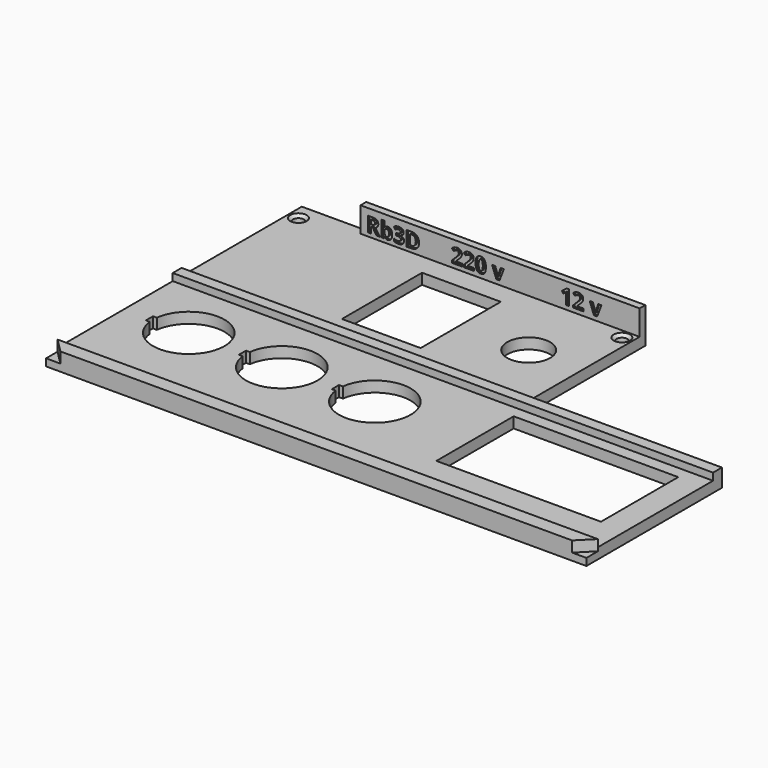
from build123d import *

# Parameters (mm, degrees)
F0_W         = 46
F0_H         = 27
F0_R         = 1.5
F0_W_2       = 22
F0_H_2       = 28
F0_R_2       = 6
F1_DEPTH     = 2
F2_DEPTH     = 10
F3_TEXT_SIZE = 5.7983598792
F4_DEPTH     = 0.5
F5_W         = 46
F5_H         = 27
F5_R         = 1.5
F5_W_2       = 22
F5_H_2       = 28
F5_R_2       = 6
F6_DEPTH     = 1
F7_SIZE      = 0.8
F9_DEPTH     = 2


# Not quite as in the source:
# - Text() gives the source's letters only with a copy of the font that has no kerning and outlines rounded to 1/6400 em; it was checked with that copy


with BuildPart() as f1:
    # F0 (on Top) → F1 (new body)
    with BuildSketch(Plane.XY):
        Polygon((0, 0), (151, 0), (151, 47.3419347727), (96, 47.3419347727), (96, 87.3419347727), (18, 87.3419347727), (18, 89.3419347727), (0, 89.3419347727), align=None)
        with BuildLine():
            ThreePointArc((8.0784325835, 28.5919347727), (28, 27.3419347727), (8.0784325835, 26.0919347727))
            Line((8.0784325835, 26.0919347727), (7, 26.0919347727))
            Line((7, 26.0919347727), (7, 28.5919347727))
            Line((7, 28.5919347727), (8.0784325835, 28.5919347727))
        make_face(mode=Mode.SUBTRACT)
        with BuildLine():
            ThreePointArc((34.0784325835, 28.5919347727), (54, 27.3419347727), (34.0784325835, 26.0919347727))
            Line((34.0784325835, 26.0919347727), (33, 26.0919347727))
            Line((33, 26.0919347727), (33, 28.5919347727))
            Line((33, 28.5919347727), (34.0784325835, 28.5919347727))
        make_face(mode=Mode.SUBTRACT)
        with BuildLine():
            ThreePointArc((60.0784325835, 28.5919347727), (80, 27.3419347727), (60.0784325835, 26.0919347727))
            Line((60.0784325835, 26.0919347727), (59, 26.0919347727))
            Line((59, 26.0919347727), (59, 28.5919347727))
            Line((59, 28.5919347727), (60.0784325835, 28.5919347727))
        make_face(mode=Mode.SUBTRACT)
        with Locations((121, 27.3419347727)):
            Rectangle(F0_W, F0_H, mode=Mode.SUBTRACT)
        with Locations((2.8, 84.6419347727)):
            Circle(F0_R, mode=Mode.SUBTRACT)
        with Locations((51, 67.3419347727)):
            Rectangle(F0_W_2, F0_H_2, mode=Mode.SUBTRACT)
        with Locations((81, 67.3419347727)):
            Circle(F0_R_2, mode=Mode.SUBTRACT)
        with Locations((93.2, 84.6419347727)):
            Circle(F0_R, mode=Mode.SUBTRACT)
    extrude(amount=F1_DEPTH)

    # F0 (on Top) → F2 (join)
    with BuildSketch(Plane.XY):
        Polygon((48, 89.3419347727), (18, 89.3419347727), (18, 87.3419347727), (96, 87.3419347727), (96, 89.3419347727), align=None)
    extrude(amount=F2_DEPTH)

    # F3 (on face) → F4 (cut)
    with BuildSketch(Plane.XZ.offset(-87.3419347727)):
        with Locations((19.5889823569, 3.9946256652)):
            Text('Rb3D', F3_TEXT_SIZE, font='Open Sans', font_style=FontStyle.BOLD, text_align=(TextAlign.LEFT, TextAlign.BOTTOM))
        with Locations((43.3194876148, 4.144287806)):
            Text('220 v', F3_TEXT_SIZE, font='Open Sans', font_style=FontStyle.BOLD, text_align=(TextAlign.LEFT, TextAlign.BOTTOM))
        with Locations((73.9085130824, 4.1421930287)):
            Text('12 v', F3_TEXT_SIZE, font='Open Sans', font_style=FontStyle.BOLD, text_align=(TextAlign.LEFT, TextAlign.BOTTOM))
    extrude(amount=-F4_DEPTH, mode=Mode.SUBTRACT)

    # F5 (on face) → F6 (join)
    with BuildSketch(Plane.XY.offset(2)):
        Polygon((0, 89.3419347727), (0, 4), (4, 0), (147, 0), (151, 4), (151, 47.3419347727), (96, 47.3419347727), (96, 87.3419347727), (18, 87.3419347727), (18, 89.3419347727), align=None)
        with BuildLine():
            Line((7, 26.0919347727), (7, 28.5919347727))
            Line((7, 28.5919347727), (8.0784325835, 28.5919347727))
            ThreePointArc((8.0784325835, 28.5919347727), (28, 27.3419347727), (8.0784325835, 26.0919347727))
            Line((8.0784325835, 26.0919347727), (7, 26.0919347727))
        make_face(mode=Mode.SUBTRACT)
        with BuildLine():
            Line((34.0784325835, 26.0919347727), (33, 26.0919347727))
            Line((33, 26.0919347727), (33, 28.5919347727))
            Line((33, 28.5919347727), (34.0784325835, 28.5919347727))
            ThreePointArc((34.0784325835, 28.5919347727), (54, 27.3419347727), (34.0784325835, 26.0919347727))
        make_face(mode=Mode.SUBTRACT)
        with BuildLine():
            Line((59, 28.5919347727), (60.0784325835, 28.5919347727))
            ThreePointArc((60.0784325835, 28.5919347727), (80, 27.3419347727), (60.0784325835, 26.0919347727))
            Line((60.0784325835, 26.0919347727), (59, 26.0919347727))
            Line((59, 26.0919347727), (59, 28.5919347727))
        make_face(mode=Mode.SUBTRACT)
        with Locations((121, 27.3419347727)):
            Rectangle(F5_W, F5_H, mode=Mode.SUBTRACT)
        with Locations((2.8, 84.6419347727)):
            Circle(F5_R, mode=Mode.SUBTRACT)
        with Locations((51, 67.3419347727)):
            Rectangle(F5_W_2, F5_H_2, mode=Mode.SUBTRACT)
        with Locations((81, 67.3419347727)):
            Circle(F5_R_2, mode=Mode.SUBTRACT)
        with Locations((93.2, 84.6419347727)):
            Circle(F5_R, mode=Mode.SUBTRACT)
    extrude(amount=F6_DEPTH)

    # F7
    f7_edges = [f1.edges().sort_by_distance(p)[0] for p in [
        (91.7, 84.641935, 3),
        (1.3, 84.641935, 3),
    ]]
    chamfer(f7_edges, length=F7_SIZE)

    # F8 (on face) → F9 (join)
    with BuildSketch(Plane.XY.offset(3)):
        Polygon((0, 47.3419347727), (0, 44.2460402846), (151, 44.2460402846), (151, 47.3419347727), (96, 47.3419347727), align=None)
        Polygon((0, 4), (4, 0), (147, 0), (151, 4), align=None)
    extrude(amount=F9_DEPTH)


solid = f1.part
